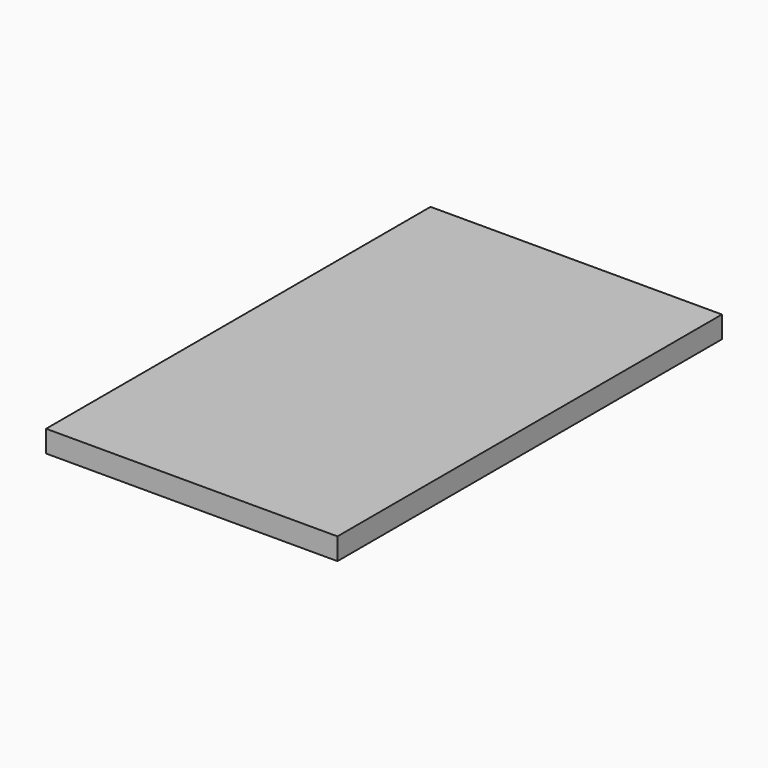
from build123d import *

# Parameters (mm, degrees)
F0_W     = 169.418
F0_H     = 279.4
F1_DEPTH = 12.7


# Not quite as in the source:
# - a feature of the source that left no trace in its solid (it failed there, or was rolled back) is left out


with BuildPart() as f1:
    # F0 (on Top) → F1 (new body)
    with BuildSketch(Plane.XY):
        Rectangle(F0_W, F0_H)
    extrude(amount=F1_DEPTH)


solid = f1.part
